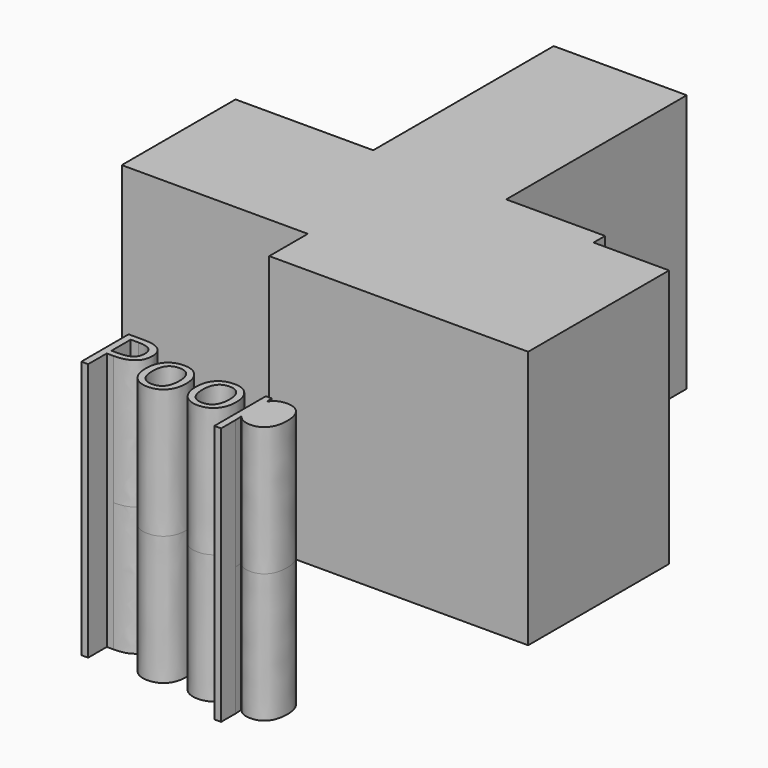
from build123d import *

# Parameters (mm, degrees)
F0_W         = 18.306851387
F0_H         = 31.0460310429
F0_TEXT_SIZE = 11.4091154602
F0_W_2       = 13.6002707295
F0_H_2       = 1.9741021097
F1_DEPTH     = 17.78


# Not quite as in the source:
# - Text() gives the source's letters only with a copy of the font that has no kerning and outlines rounded to 1/6400 em; it was checked with that copy


with BuildPart() as f1:
    # F0 (on Top) → F1 (new body, symmetric)
    with BuildSketch(Plane.XY):
        Polygon((-5.3398390301, 6.6365879029), (-30.5835790932, 6.6365879029), (-30.5835790932, 0), (5.0467923284, 0), (5.0467923284, 24.2371428758), (-5.3398390301, 24.2371428758), align=None)
        with Locations((-28.0935354531, 41.7342605069)):
            Rectangle(F0_W, F0_H)
        with Locations((-32.1347601712, -31.7949317396)):
            Text('Poop', F0_TEXT_SIZE, font='Open Sans', text_align=(TextAlign.LEFT, TextAlign.BOTTOM))
        with Locations((-12.1399743948, 25.2241939306)):
            Rectangle(F0_W_2, F0_H_2)
        Polygon((-30.5835790932, 6.6365879029), (-30.5835790932, 24.2371428758), (-37.2469611466, 24.2371428758), (-37.2469611466, 26.2112449855), (-56.1897531152, 26.2112449855), (-56.1897531152, 6.6365879029), align=None)
        Polygon((-18.9401097596, 24.2371428758), (-30.5835790932, 24.2371428758), (-30.5835790932, 6.6365879029), (-5.3398390301, 6.6365879029), (-5.3398390301, 24.2371428758), align=None)
        Polygon((-37.2469611466, 24.2371428758), (-30.5835790932, 24.2371428758), (-18.9401097596, 24.2371428758), (-18.9401097596, 26.2112449855), (-37.2469611466, 26.2112449855), align=None)
        with BuildLine():
            add(Edge.make_bspline(
                [(-6.532883346, -26.9727977834), (-6.9812259301, -26.3631231759), (-7.7941254066, -26.3631231759)],
                knots=[0, 0, 0, 1, 1, 1], degree=2))
            add(Edge.make_bspline(
                [(-7.7941254066, -26.3631231759), (-8.7300294092, -26.3631231759), (-9.1480665303, -26.8809900574)],
                knots=[0, 0, 0, 1, 1, 1], degree=2))
            add(Edge.make_bspline(
                [(-9.1480665303, -26.8809900574), (-9.5661036515, -27.3988569388), (-9.5767996972, -28.5308551134)],
                knots=[0, 0, 0, 1, 1, 1], degree=2))
            Line((-9.5767996972, -28.5308551134), (-9.5767996972, -28.7358626568))
            add(Edge.make_bspline(
                [(-9.5767996972, -28.7358626568), (-9.5767996972, -30.0229534947), (-9.1480665303, -30.5773651991)],
                knots=[0, 0, 0, 1, 1, 1], degree=2))
            add(Edge.make_bspline(
                [(-9.1480665303, -30.5773651991), (-8.7193333634, -31.1317769034), (-7.7727333151, -31.1317769034)],
                knots=[0, 0, 0, 1, 1, 1], degree=2))
            add(Edge.make_bspline(
                [(-7.7727333151, -31.1317769034), (-6.9812259301, -31.1317769034), (-6.532883346, -30.490905496)],
                knots=[0, 0, 0, 1, 1, 1], degree=2))
            add(Edge.make_bspline(
                [(-6.532883346, -30.490905496), (-6.0845407619, -29.8500340885), (-6.0845407619, -28.7251666111)],
                knots=[0, 0, 0, 1, 1, 1], degree=2))
            add(Edge.make_bspline(
                [(-6.0845407619, -28.7251666111), (-6.0845407619, -27.5824723908), (-6.532883346, -26.9727977834)],
                knots=[0, 0, 0, 1, 1, 1], degree=2))
        make_face()
    extrude(amount=F1_DEPTH, both=True)


solid = f1.part
